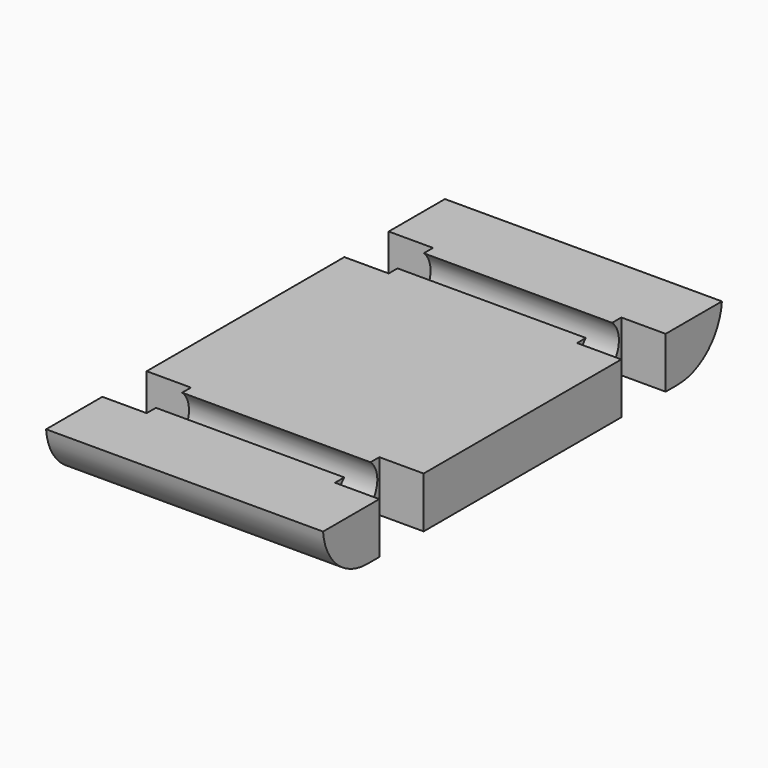
from build123d import *

# Parameters (mm, degrees)
F1_DEPTH    = 2.3
F2_R        = 2.25
F3_DEPTH    = 25
F4_T1_DEPTH = 49.9198715888


# Not quite as in the source:
# - a fillet or chamfer that OpenCascade refuses, or shapes differently, is made with other operations: its cross-section is extruded or revolved along the edge and cut away or added


with BuildPart() as f1:
    # F0 (on Top) → F1 (new body, symmetric)
    with BuildSketch(Plane.XY):
        Polygon((12.5, 22.5), (-12.5, 22.5), (-12.5, 16.1530176364), (-8.5, 16.1530176364), (-8.5, 11.1530176364), (-12.5, 11.1530176364), (-12.5, -11.1530176364), (-8.5, -11.1530176364), (-8.5, -16.1530176364), (-12.5, -16.1530176364), (-12.5, -22.5), (12.5, -22.5), (12.5, -16.1530176364), (8.5, -16.1530176364), (8.5, -11.1530176364), (12.5, -11.1530176364), (12.5, 11.1530176364), (8.5, 11.1530176364), (8.5, 16.1530176364), (12.5, 16.1530176364), align=None)
    extrude(amount=F1_DEPTH, both=True)

    # F2 (on face) → F3 (cut)
    with BuildSketch(Plane.YZ.offset(8.5)):
        with Locations((-13.6288348585, 0.6045123446)):
            Circle(F2_R)
        with Locations((13.6288348585, 0.6045123446)):
            Circle(F2_R)
    extrude(amount=-F3_DEPTH, mode=Mode.SUBTRACT)

    # F4: fillet of radius 5 on 2 edges, made by hand

    # F4_s2 → F4_t1 (cut)
    with BuildSketch(Plane.YZ.offset(-24.9599357944)):
        with BuildLine():
            ThreePointArc((-22.5, 2.3), (-20.9071906738, -0.9742346142), (-17.5160256822, -2.3))
            Line((-17.5160256822, -2.3), (-22.5, -2.3))
            Line((-22.5, -2.3), (-22.5, 2.3))
        make_face()
        with BuildLine():
            ThreePointArc((22.5, 2.3), (20.9071906738, -0.9742346142), (17.5160256822, -2.3))
            Line((17.5160256822, -2.3), (22.5, -2.3))
            Line((22.5, -2.3), (22.5, 2.3))
        make_face()
    extrude(amount=F4_T1_DEPTH, mode=Mode.SUBTRACT)


solid = f1.part
